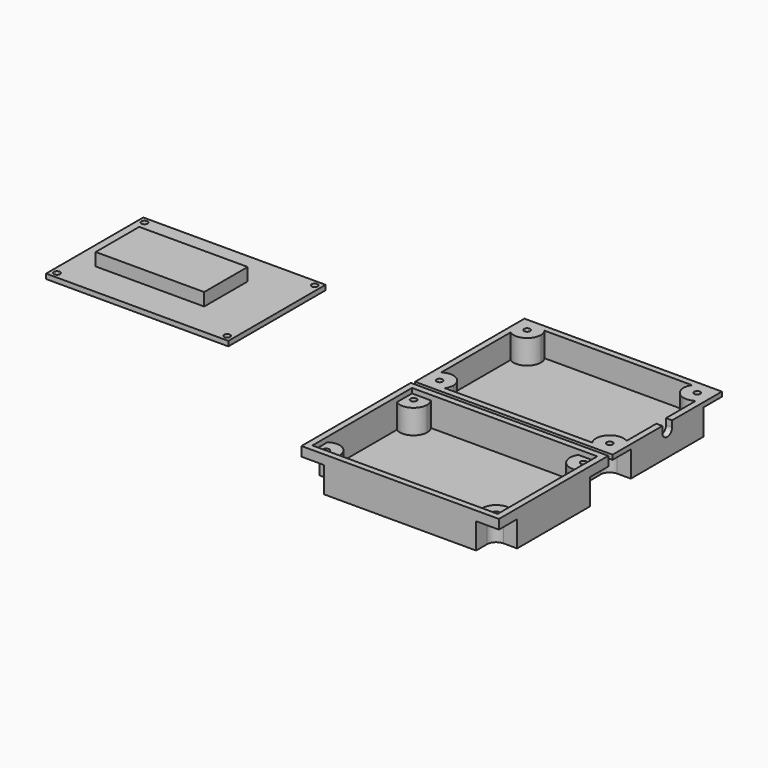
from build123d import *

# Parameters (mm, degrees)
F0_W      = 60
F0_H      = 40
F0_R      = 1
F1_DEPTH  = 1.6
F3_W      = 35.7
F3_H      = 17.9
F4_DEPTH  = 4.2
F5_W      = 65
F5_H      = 45
F5_R      = 1
F6_DEPTH  = 2
F7_R      = 1
F8_DEPTH  = 8
F9_W      = 65
F9_H      = 45
F9_R      = 1
F10_DEPTH = 2
F11_R     = 1
F12_DEPTH = 8
F13_W     = 65
F13_H     = 45
F13_W_2   = 61
F13_H_2   = 41
F14_DEPTH = 1.6
F16_DEPTH = 8.5
F18_DEPTH = 8.5
F20_DEPTH = 25.4


with BuildPart() as f1:
    # F0 (on Top) → F1 (new body)
    with BuildSketch(Plane.XY):
        with Locations((-71.7097583413, 11.8171558529)):
            Rectangle(F0_W, F0_H)
        with Locations((-99.7097583413, -6.1828441471)):
            Circle(F0_R, mode=Mode.SUBTRACT)
        with Locations((-43.7097583413, -6.1828441471)):
            Circle(F0_R, mode=Mode.SUBTRACT)
        with Locations((-99.7097583413, 29.8171558529)):
            Circle(F0_R, mode=Mode.SUBTRACT)
        with Locations((-43.7097583413, 29.8171558529)):
            Circle(F0_R, mode=Mode.SUBTRACT)
    extrude(amount=F1_DEPTH)

    # F3 (on face) → F4 (join)
    with BuildSketch(Plane.XY.offset(1.6)):
        with Locations((-76.3597583413, 11.8171558529)):
            Rectangle(F3_W, F3_H)
    extrude(amount=F4_DEPTH)


with BuildPart() as f6:
    # F5 (on Top) → F6 (new body)
    with BuildSketch(Plane.XY):
        with Locations((52.5504697859, 13.9392828941)):
            Rectangle(F5_W, F5_H)
        with Locations((24.5504697859, -4.0607171059)):
            Circle(F5_R, mode=Mode.SUBTRACT)
        with Locations((80.5504697859, -4.0607171059)):
            Circle(F5_R, mode=Mode.SUBTRACT)
        with Locations((24.5504697859, 31.9392828941)):
            Circle(F5_R, mode=Mode.SUBTRACT)
        with Locations((80.5504697859, 31.9392828941)):
            Circle(F5_R, mode=Mode.SUBTRACT)
    extrude(amount=F6_DEPTH)

    # F7 (on face) → F8 (join)
    with BuildSketch(Plane.XY.offset(2)):
        with BuildLine():
            Line((22.0504697859, 34.4392828941), (28.2921271727, 34.4392828941))
            ThreePointArc((28.2921271727, 34.4392828941), (26.6717901295, 35.9079098607), (24.5504697859, 36.4392828941))
            ThreePointArc((24.5504697859, 36.4392828941), (21.3684892706, 35.1212634095), (20.0504697859, 31.9392828941))
            ThreePointArc((20.0504697859, 31.9392828941), (20.5818428193, 29.8179625506), (22.0504697859, 28.1976255074))
            Line((22.0504697859, 28.1976255074), (22.0504697859, 34.4392828941))
        make_face()
        with BuildLine():
            ThreePointArc((24.5504697859, 36.4392828941), (26.6717901295, 35.9079098607), (28.2921271727, 34.4392828941))
            Line((28.2921271727, 34.4392828941), (76.8088123992, 34.4392828941))
            ThreePointArc((76.8088123992, 34.4392828941), (78.4291494424, 35.9079098607), (80.5504697859, 36.4392828941))
            Line((80.5504697859, 36.4392828941), (24.5504697859, 36.4392828941))
        make_face()
        with BuildLine():
            Line((22.0504697859, -0.3190597191), (22.0504697859, 28.1976255074))
            ThreePointArc((22.0504697859, 28.1976255074), (20.5818428193, 29.8179625506), (20.0504697859, 31.9392828941))
            Line((20.0504697859, 31.9392828941), (20.0504697859, -4.060717062))
            ThreePointArc((20.0504697859, -4.060717062), (20.5818428297, -1.939396743), (22.0504697859, -0.3190597191))
        make_face()
        with BuildLine():
            ThreePointArc((20.0504697859, 31.9392828941), (21.3684892706, 35.1212634095), (24.5504697859, 36.4392828941))
            Line((24.5504697859, 36.4392828941), (20.0504697859, 36.4392828941))
            Line((20.0504697859, 36.4392828941), (20.0504697859, 31.9392828941))
        make_face()
        with BuildLine():
            ThreePointArc((80.5504697859, 36.4392828941), (78.4291494424, 35.9079098607), (76.8088123992, 34.4392828941))
            Line((76.8088123992, 34.4392828941), (83.0504697859, 34.4392828941))
            Line((83.0504697859, 34.4392828941), (83.0504697859, 28.1976255074))
            ThreePointArc((83.0504697859, 28.1976255074), (84.5190967525, 29.8179625506), (85.0504697859, 31.9392828941))
            ThreePointArc((85.0504697859, 31.9392828941), (83.7324503013, 35.1212634095), (80.5504697859, 36.4392828941))
        make_face()
        with BuildLine():
            Line((22.0504697859, -6.5607171059), (22.0504697859, -0.3190597191))
            ThreePointArc((22.0504697859, -0.3190597191), (20.5818428297, -1.939396743), (20.0504697859, -4.060717062))
            ThreePointArc((20.0504697859, -4.060717062), (21.3684892551, -7.2426976057), (24.5504697859, -8.5607171059))
            ThreePointArc((24.5504697859, -8.5607171059), (26.6717901295, -8.0293440725), (28.2921271727, -6.5607171059))
            Line((28.2921271727, -6.5607171059), (22.0504697859, -6.5607171059))
        make_face()
        with BuildLine():
            Line((85.0504697859, 36.4392828941), (80.5504697859, 36.4392828941))
            ThreePointArc((80.5504697859, 36.4392828941), (83.7324503013, 35.1212634095), (85.0504697859, 31.9392828941))
            Line((85.0504697859, 31.9392828941), (85.0504697859, 36.4392828941))
        make_face()
        with BuildLine():
            ThreePointArc((85.0504697859, 31.9392828941), (84.5190967525, 29.8179625506), (83.0504697859, 28.1976255074))
            Line((83.0504697859, 28.1976255074), (83.0504697859, -0.3190597191))
            ThreePointArc((83.0504697859, -0.3190597191), (84.5190967525, -1.9393967623), (85.0504697859, -4.0607171059))
            Line((85.0504697859, -4.0607171059), (85.0504697859, 31.9392828941))
        make_face()
        with BuildLine():
            ThreePointArc((24.5504697859, -8.5607171059), (21.3684892551, -7.2426976057), (20.0504697859, -4.060717062))
            Line((20.0504697859, -4.060717062), (20.0504697859, -8.5607171059))
            Line((20.0504697859, -8.5607171059), (24.5504697859, -8.5607171059))
        make_face()
        with BuildLine():
            ThreePointArc((85.0504697859, -4.0607171059), (84.5190967525, -1.9393967623), (83.0504697859, -0.3190597191))
            Line((83.0504697859, -0.3190597191), (83.0504697859, -6.5607171059))
            Line((83.0504697859, -6.5607171059), (76.8088123992, -6.5607171059))
            ThreePointArc((76.8088123992, -6.5607171059), (78.4291494424, -8.0293440725), (80.5504697859, -8.5607171059))
            ThreePointArc((80.5504697859, -8.5607171059), (83.7324503013, -7.2426976212), (85.0504697859, -4.0607171059))
        make_face()
        with BuildLine():
            ThreePointArc((28.2921271727, -6.5607171059), (26.6717901295, -8.0293440725), (24.5504697859, -8.5607171059))
            Line((24.5504697859, -8.5607171059), (80.5504697859, -8.5607171059))
            ThreePointArc((80.5504697859, -8.5607171059), (78.4291494424, -8.0293440725), (76.8088123992, -6.5607171059))
            Line((76.8088123992, -6.5607171059), (28.2921271727, -6.5607171059))
        make_face()
        with BuildLine():
            Line((85.0504697859, -8.5607171059), (85.0504697859, -4.0607171059))
            ThreePointArc((85.0504697859, -4.0607171059), (83.7324503013, -7.2426976212), (80.5504697859, -8.5607171059))
            Line((80.5504697859, -8.5607171059), (85.0504697859, -8.5607171059))
        make_face()
        with BuildLine():
            ThreePointArc((22.0504697859, 28.1976255074), (26.6717901295, 27.9706559275), (29.0504697859, 31.9392828941))
            ThreePointArc((29.0504697859, 31.9392828941), (28.856712826, 33.2455259342), (28.2921271727, 34.4392828941))
            Line((28.2921271727, 34.4392828941), (22.0504697859, 34.4392828941))
            Line((22.0504697859, 34.4392828941), (22.0504697859, 28.1976255074))
        make_face()
        with Locations((24.5504697859, 31.9392828941)):
            Circle(F7_R, mode=Mode.SUBTRACT)
        with BuildLine():
            ThreePointArc((29.0504697859, -4.0607171059), (26.6717901295, -0.0920901393), (22.0504697859, -0.3190597191))
            Line((22.0504697859, -0.3190597191), (22.0504697859, -6.5607171059))
            Line((22.0504697859, -6.5607171059), (28.2921271727, -6.5607171059))
            ThreePointArc((28.2921271727, -6.5607171059), (28.856712826, -5.3669601459), (29.0504697859, -4.0607171059))
        make_face()
        with Locations((24.5504697859, -4.0607171059)):
            Circle(F7_R, mode=Mode.SUBTRACT)
        with BuildLine():
            Line((83.0504697859, -6.5607171059), (83.0504697859, -0.3190597191))
            ThreePointArc((83.0504697859, -0.3190597191), (77.3684892706, -0.8787365905), (76.8088123992, -6.5607171059))
            Line((76.8088123992, -6.5607171059), (83.0504697859, -6.5607171059))
        make_face()
        with Locations((80.5504697859, -4.0607171059)):
            Circle(F7_R, mode=Mode.SUBTRACT)
        with BuildLine():
            Line((83.0504697859, 34.4392828941), (76.8088123992, 34.4392828941))
            ThreePointArc((76.8088123992, 34.4392828941), (77.3684892706, 28.7573023788), (83.0504697859, 28.1976255074))
            Line((83.0504697859, 28.1976255074), (83.0504697859, 34.4392828941))
        make_face()
        with Locations((80.5504697859, 31.9392828941)):
            Circle(F7_R, mode=Mode.SUBTRACT)
    extrude(amount=F8_DEPTH)

    # F17 (on face) → F18 (cut)
    with BuildSketch(Plane(origin=(0, 0, 0), x_dir=(1, 0, 0), z_dir=(0, 0, -1))):
        with BuildLine():
            ThreePointArc((80.5504697859, 1.0607171059), (82.6717901295, 1.9393967623), (83.5504697859, 4.0607171059))
            ThreePointArc((83.5504697859, 4.0607171059), (80.5504697859, 7.0607171059), (77.5504697859, 4.0607171059))
            ThreePointArc((77.5504697859, 4.0607171059), (78.4291494424, 1.9393967623), (80.5504697859, 1.0607171059))
        make_face()
        with BuildLine():
            ThreePointArc((77.5504697859, -31.9392828941), (80.5504697859, -34.9392828941), (83.5504697859, -31.9392828941))
            ThreePointArc((83.5504697859, -31.9392828941), (82.6717901295, -29.8179625506), (80.5504697859, -28.9392828941))
            ThreePointArc((80.5504697859, -28.9392828941), (78.4291494424, -29.8179625506), (77.5504697859, -31.9392828941))
        make_face()
        with BuildLine():
            ThreePointArc((24.5504697859, 1.0607171059), (26.6717901295, 1.9393967623), (27.5504697859, 4.0607171059))
            ThreePointArc((27.5504697859, 4.0607171059), (22.4291494424, 6.1820374494), (24.5504697859, 1.0607171059))
        make_face()
        with BuildLine():
            ThreePointArc((24.5504697859, -28.9392828941), (22.4291494424, -34.0606032377), (27.5504697859, -31.9392828941))
            ThreePointArc((27.5504697859, -31.9392828941), (26.6717901295, -29.8179625506), (24.5504697859, -28.9392828941))
        make_face()
        with BuildLine():
            ThreePointArc((77.5504697859, 4.0607171059), (80.5504697859, 7.0607171059), (83.5504697859, 4.0607171059))
            ThreePointArc((83.5504697859, 4.0607171059), (82.6717901295, 1.9393967623), (80.5504697859, 1.0607171059))
            Line((80.5504697859, 1.0607171059), (85.0504697859, 1.0607171059))
            Line((85.0504697859, 1.0607171059), (85.0504697859, 8.5607171059))
            Line((85.0504697859, 8.5607171059), (77.5504697859, 8.5607171059))
            Line((77.5504697859, 8.5607171059), (77.5504697859, 4.0607171059))
        make_face()
        with BuildLine():
            Line((85.0504697859, -36.4392828941), (85.0504697859, -28.9392828941))
            Line((85.0504697859, -28.9392828941), (80.5504697859, -28.9392828941))
            ThreePointArc((80.5504697859, -28.9392828941), (82.6717901295, -29.8179625506), (83.5504697859, -31.9392828941))
            ThreePointArc((83.5504697859, -31.9392828941), (80.5504697859, -34.9392828941), (77.5504697859, -31.9392828941))
            Line((77.5504697859, -31.9392828941), (77.5504697859, -36.4392828941))
            Line((77.5504697859, -36.4392828941), (85.0504697859, -36.4392828941))
        make_face()
        with BuildLine():
            Line((27.5504697859, 4.0607171059), (27.5504697859, 8.5607171059))
            Line((27.5504697859, 8.5607171059), (20.0504697859, 8.5607171059))
            Line((20.0504697859, 8.5607171059), (20.0504697859, 1.0607171059))
            Line((20.0504697859, 1.0607171059), (24.5504697859, 1.0607171059))
            ThreePointArc((24.5504697859, 1.0607171059), (22.4291494424, 6.1820374494), (27.5504697859, 4.0607171059))
        make_face()
        with BuildLine():
            Line((24.5504697859, -28.9392828941), (20.0504697859, -28.9392828941))
            Line((20.0504697859, -28.9392828941), (20.0504697859, -36.4392828941))
            Line((20.0504697859, -36.4392828941), (27.5504697859, -36.4392828941))
            Line((27.5504697859, -36.4392828941), (27.5504697859, -31.9392828941))
            ThreePointArc((27.5504697859, -31.9392828941), (22.4291494424, -34.0606032377), (24.5504697859, -28.9392828941))
        make_face()
    extrude(amount=-F18_DEPTH, mode=Mode.SUBTRACT)

    # F19 (on face) → F20 (cut)
    with BuildSketch(Plane.YZ.offset(85.0504697859)):
        with BuildLine():
            ThreePointArc((13.9392828941, 10), (12.5250693318, 9.4142135624), (11.9392828941, 8))
            ThreePointArc((11.9392828941, 8), (13.9392828941, 6), (15.9392828941, 8))
            ThreePointArc((15.9392828941, 8), (15.3534964565, 9.4142135624), (13.9392828941, 10))
        make_face()
        with BuildLine():
            ThreePointArc((13.9392828941, 10), (15.3534964565, 9.4142135624), (15.9392828941, 8))
            Line((15.9392828941, 8), (15.9392828941, 10))
            Line((15.9392828941, 10), (13.9392828941, 10))
        make_face()
        with BuildLine():
            Line((11.9392828941, 10), (11.9392828941, 8))
            ThreePointArc((11.9392828941, 8), (12.5250693318, 9.4142135624), (13.9392828941, 10))
            Line((13.9392828941, 10), (11.9392828941, 10))
        make_face()
    extrude(amount=-F20_DEPTH, mode=Mode.SUBTRACT)


with BuildPart() as f10:
    # F9 (on Top) → F10 (new body)
    with BuildSketch(Plane.XY):
        with Locations((54.0033790469, -34.6341663599)):
            Rectangle(F9_W, F9_H)
        with Locations((26.0033790469, -52.6341663599)):
            Circle(F9_R, mode=Mode.SUBTRACT)
        with Locations((82.0033790469, -52.6341663599)):
            Circle(F9_R, mode=Mode.SUBTRACT)
        with Locations((26.0033790469, -16.6341663599)):
            Circle(F9_R, mode=Mode.SUBTRACT)
        with Locations((82.0033790469, -16.6341663599)):
            Circle(F9_R, mode=Mode.SUBTRACT)
    extrude(amount=F10_DEPTH)

    # F11 (on face) → F12 (join)
    with BuildSketch(Plane.XY.offset(2)):
        with BuildLine():
            Line((23.5033790469, -14.1341663599), (29.7450364337, -14.1341663599))
            ThreePointArc((29.7450364337, -14.1341663599), (28.1246993905, -12.6655393933), (26.0033790469, -12.1341663599))
            ThreePointArc((26.0033790469, -12.1341663599), (22.8213985316, -13.4521858446), (21.5033790469, -16.6341663599))
            ThreePointArc((21.5033790469, -16.6341663599), (22.0347520803, -18.7554867035), (23.5033790469, -20.3758237467))
            Line((23.5033790469, -20.3758237467), (23.5033790469, -14.1341663599))
        make_face()
        with BuildLine():
            ThreePointArc((26.0033790469, -12.1341663599), (28.1246993905, -12.6655393933), (29.7450364337, -14.1341663599))
            Line((29.7450364337, -14.1341663599), (78.2617216601, -14.1341663599))
            ThreePointArc((78.2617216601, -14.1341663599), (79.8820586955, -12.6655393975), (82.003379029, -12.1341663599))
            Line((82.003379029, -12.1341663599), (26.0033790469, -12.1341663599))
        make_face()
        with BuildLine():
            Line((23.5033790469, -48.8925089731), (23.5033790469, -20.3758237467))
            ThreePointArc((23.5033790469, -20.3758237467), (22.0347520803, -18.7554867035), (21.5033790469, -16.6341663599))
            Line((21.5033790469, -16.6341663599), (21.5033790469, -52.6341663599))
            ThreePointArc((21.5033790469, -52.6341663599), (22.0347520803, -50.5128460163), (23.5033790469, -48.8925089731))
        make_face()
        with BuildLine():
            ThreePointArc((21.5033790469, -16.6341663599), (22.8213985316, -13.4521858446), (26.0033790469, -12.1341663599))
            Line((26.0033790469, -12.1341663599), (21.5033790469, -12.1341663599))
            Line((21.5033790469, -12.1341663599), (21.5033790469, -16.6341663599))
        make_face()
        with BuildLine():
            ThreePointArc((82.003379029, -12.1341663599), (79.8820586955, -12.6655393975), (78.2617216601, -14.1341663599))
            Line((78.2617216601, -14.1341663599), (84.5033790469, -14.1341663599))
            Line((84.5033790469, -14.1341663599), (84.5033790469, -20.3758237467))
            ThreePointArc((84.5033790469, -20.3758237467), (85.9720060135, -18.7554867035), (86.5033790469, -16.6341663599))
            ThreePointArc((86.5033790469, -16.6341663599), (85.1853595559, -13.4521858382), (82.003379029, -12.1341663599))
        make_face()
        with BuildLine():
            Line((23.5033790469, -55.1341663599), (23.5033790469, -48.8925089731))
            ThreePointArc((23.5033790469, -48.8925089731), (22.0347520803, -50.5128460163), (21.5033790469, -52.6341663599))
            ThreePointArc((21.5033790469, -52.6341663599), (22.8213985316, -55.8161468752), (26.0033790469, -57.1341663599))
            ThreePointArc((26.0033790469, -57.1341663599), (28.1246993905, -56.6027933265), (29.7450364337, -55.1341663599))
            Line((29.7450364337, -55.1341663599), (23.5033790469, -55.1341663599))
        make_face()
        with BuildLine():
            Line((86.5033790469, -12.1341663599), (82.003379029, -12.1341663599))
            ThreePointArc((82.003379029, -12.1341663599), (85.1853595559, -13.4521858382), (86.5033790469, -16.6341663599))
            Line((86.5033790469, -16.6341663599), (86.5033790469, -12.1341663599))
        make_face()
        with BuildLine():
            ThreePointArc((86.5033790469, -16.6341663599), (85.9720060135, -18.7554867035), (84.5033790469, -20.3758237467))
            Line((84.5033790469, -20.3758237467), (84.5033790469, -48.8925089731))
            ThreePointArc((84.5033790469, -48.8925089731), (85.9720060135, -50.5128460163), (86.5033790469, -52.6341663599))
            Line((86.5033790469, -52.6341663599), (86.5033790469, -16.6341663599))
        make_face()
        with BuildLine():
            ThreePointArc((26.0033790469, -57.1341663599), (22.8213985316, -55.8161468752), (21.5033790469, -52.6341663599))
            Line((21.5033790469, -52.6341663599), (21.5033790469, -57.1341663599))
            Line((21.5033790469, -57.1341663599), (26.0033790469, -57.1341663599))
        make_face()
        with BuildLine():
            ThreePointArc((86.5033790469, -52.6341663599), (85.9720060135, -50.5128460163), (84.5033790469, -48.8925089731))
            Line((84.5033790469, -48.8925089731), (84.5033790469, -55.1341663599))
            Line((84.5033790469, -55.1341663599), (78.2617216601, -55.1341663599))
            ThreePointArc((78.2617216601, -55.1341663599), (79.8820587034, -56.6027933265), (82.0033790469, -57.1341663599))
            ThreePointArc((82.0033790469, -57.1341663599), (85.1853595623, -55.8161468752), (86.5033790469, -52.6341663599))
        make_face()
        with BuildLine():
            ThreePointArc((29.7450364337, -55.1341663599), (28.1246993905, -56.6027933265), (26.0033790469, -57.1341663599))
            Line((26.0033790469, -57.1341663599), (82.0033790469, -57.1341663599))
            ThreePointArc((82.0033790469, -57.1341663599), (79.8820587034, -56.6027933265), (78.2617216601, -55.1341663599))
            Line((78.2617216601, -55.1341663599), (29.7450364337, -55.1341663599))
        make_face()
        with BuildLine():
            Line((86.5033790469, -57.1341663599), (86.5033790469, -52.6341663599))
            ThreePointArc((86.5033790469, -52.6341663599), (85.1853595623, -55.8161468752), (82.0033790469, -57.1341663599))
            Line((82.0033790469, -57.1341663599), (86.5033790469, -57.1341663599))
        make_face()
        with BuildLine():
            ThreePointArc((30.5033790469, -52.6341663599), (28.1246993905, -48.6655393933), (23.5033790469, -48.8925089731))
            Line((23.5033790469, -48.8925089731), (23.5033790469, -55.1341663599))
            Line((23.5033790469, -55.1341663599), (29.7450364337, -55.1341663599))
            ThreePointArc((29.7450364337, -55.1341663599), (30.309622087, -53.9404094), (30.5033790469, -52.6341663599))
        make_face()
        with Locations((26.0033790469, -52.6341663599)):
            Circle(F11_R, mode=Mode.SUBTRACT)
        with BuildLine():
            ThreePointArc((26.003379073, -12.1341663599), (28.124699402, -12.6655393994), (29.7450364337, -14.1341663599))
            Line((29.7450364337, -14.1341663599), (78.2617216601, -14.1341663599))
            ThreePointArc((78.2617216601, -14.1341663599), (79.8820586955, -12.6655393975), (82.003379029, -12.1341663599))
            Line((82.003379029, -12.1341663599), (26.003379073, -12.1341663599))
        make_face()
        with BuildLine():
            ThreePointArc((23.5033790469, -20.3758237467), (28.1246993905, -20.6027933265), (30.5033790469, -16.6341663599))
            ThreePointArc((30.5033790469, -16.6341663599), (30.309622087, -15.3279233198), (29.7450364337, -14.1341663599))
            Line((29.7450364337, -14.1341663599), (23.5033790469, -14.1341663599))
            Line((23.5033790469, -14.1341663599), (23.5033790469, -20.3758237467))
        make_face()
        with Locations((26.0033790469, -16.6341663599)):
            Circle(F11_R, mode=Mode.SUBTRACT)
        with BuildLine():
            Line((84.5033790469, -14.1341663599), (78.2617216601, -14.1341663599))
            ThreePointArc((78.2617216601, -14.1341663599), (78.8213985316, -19.8161468752), (84.5033790469, -20.3758237467))
            Line((84.5033790469, -20.3758237467), (84.5033790469, -14.1341663599))
        make_face()
        with Locations((82.0033790469, -16.6341663599)):
            Circle(F11_R, mode=Mode.SUBTRACT)
        with BuildLine():
            Line((84.5033790469, -55.1341663599), (84.5033790469, -48.8925089731))
            ThreePointArc((84.5033790469, -48.8925089731), (78.8213985316, -49.4521858446), (78.2617216601, -55.1341663599))
            Line((78.2617216601, -55.1341663599), (84.5033790469, -55.1341663599))
        make_face()
        with Locations((82.0033790469, -52.6341663599)):
            Circle(F11_R, mode=Mode.SUBTRACT)
        with BuildLine():
            Line((23.5033790469, -14.1341663599), (29.7450364337, -14.1341663599))
            ThreePointArc((29.7450364337, -14.1341663599), (28.124699402, -12.6655393994), (26.003379073, -12.1341663599))
            ThreePointArc((26.003379073, -12.1341663599), (22.8213985408, -13.4521858354), (21.5033790469, -16.6341663599))
            ThreePointArc((21.5033790469, -16.6341663599), (22.0347520803, -18.7554867035), (23.5033790469, -20.3758237467))
            Line((23.5033790469, -20.3758237467), (23.5033790469, -14.1341663599))
        make_face()
    extrude(amount=F12_DEPTH)

    # F13 (on face) → F14 (join)
    with BuildSketch(Plane.XY.offset(10)):
        with Locations((54.0033790469, -34.6341663599)):
            Rectangle(F13_W, F13_H)
        with Locations((54.0033790469, -34.6341663599)):
            Rectangle(F13_W_2, F13_H_2, mode=Mode.SUBTRACT)
    extrude(amount=F14_DEPTH)

    # F15 (on face) → F16 (cut)
    with BuildSketch(Plane(origin=(0, 0, 0), x_dir=(1, 0, 0), z_dir=(0, 0, -1))):
        with BuildLine():
            ThreePointArc((82.0033790469, 49.6341663599), (84.1246993905, 50.5128460163), (85.0033790469, 52.6341663599))
            ThreePointArc((85.0033790469, 52.6341663599), (82.0033790469, 55.6341663599), (79.0033790469, 52.6341663599))
            ThreePointArc((79.0033790469, 52.6341663599), (79.8820587034, 50.5128460163), (82.0033790469, 49.6341663599))
        make_face()
        with BuildLine():
            ThreePointArc((79.0033790469, 16.6341663599), (82.0033790469, 13.6341663599), (85.0033790469, 16.6341663599))
            ThreePointArc((85.0033790469, 16.6341663599), (84.1246993905, 18.7554867035), (82.0033790469, 19.6341663599))
            ThreePointArc((82.0033790469, 19.6341663599), (79.8820587034, 18.7554867035), (79.0033790469, 16.6341663599))
        make_face()
        with BuildLine():
            ThreePointArc((26.0033790469, 49.6341663599), (28.1246993905, 50.5128460163), (29.0033790469, 52.6341663599))
            ThreePointArc((29.0033790469, 52.6341663599), (23.8820587034, 54.7554867035), (26.0033790469, 49.6341663599))
        make_face()
        with BuildLine():
            ThreePointArc((26.0033790469, 19.6341663599), (23.8820587034, 14.5128460163), (29.0033790469, 16.6341663599))
            ThreePointArc((29.0033790469, 16.6341663599), (28.1246993905, 18.7554867035), (26.0033790469, 19.6341663599))
        make_face()
        with BuildLine():
            Line((29.0033790469, 52.6341663599), (29.0033790469, 57.1341663599))
            Line((29.0033790469, 57.1341663599), (21.5033790469, 57.1341663599))
            Line((21.5033790469, 57.1341663599), (21.5033790469, 49.6341663599))
            Line((21.5033790469, 49.6341663599), (26.0033790469, 49.6341663599))
            ThreePointArc((26.0033790469, 49.6341663599), (23.8820587034, 54.7554867035), (29.0033790469, 52.6341663599))
        make_face()
        with BuildLine():
            Line((26.0033790469, 19.6341663599), (21.5033790469, 19.6341663599))
            Line((21.5033790469, 19.6341663599), (21.5033790469, 12.1341663599))
            Line((21.5033790469, 12.1341663599), (29.0033790469, 12.1341663599))
            Line((29.0033790469, 12.1341663599), (29.0033790469, 16.6341663599))
            ThreePointArc((29.0033790469, 16.6341663599), (23.8820587034, 14.5128460163), (26.0033790469, 19.6341663599))
        make_face()
        with BuildLine():
            Line((86.5033790469, 12.1341663599), (86.5033790469, 19.6341663599))
            Line((86.5033790469, 19.6341663599), (82.0033790469, 19.6341663599))
            ThreePointArc((82.0033790469, 19.6341663599), (84.1246993905, 18.7554867035), (85.0033790469, 16.6341663599))
            ThreePointArc((85.0033790469, 16.6341663599), (82.0033790469, 13.6341663599), (79.0033790469, 16.6341663599))
            Line((79.0033790469, 16.6341663599), (79.0033790469, 12.1341663599))
            Line((79.0033790469, 12.1341663599), (86.5033790469, 12.1341663599))
        make_face()
        with BuildLine():
            ThreePointArc((79.0033790469, 52.6341663599), (82.0033790469, 55.6341663599), (85.0033790469, 52.6341663599))
            ThreePointArc((85.0033790469, 52.6341663599), (84.1246993905, 50.5128460163), (82.0033790469, 49.6341663599))
            Line((82.0033790469, 49.6341663599), (86.5033790469, 49.6341663599))
            Line((86.5033790469, 49.6341663599), (86.5033790469, 57.1341663599))
            Line((86.5033790469, 57.1341663599), (79.0033790469, 57.1341663599))
            Line((79.0033790469, 57.1341663599), (79.0033790469, 52.6341663599))
        make_face()
    extrude(amount=-F16_DEPTH, mode=Mode.SUBTRACT)


solid = Compound([f1.part, f6.part, f10.part])
